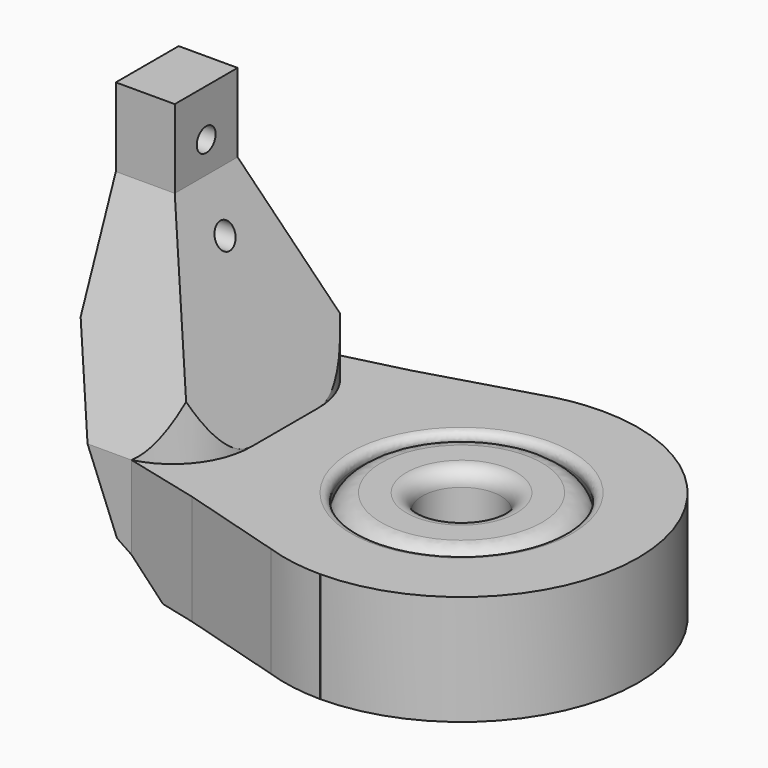
from build123d import *

# Parameters (mm, degrees)
F3_R         = 3
F4_R         = 1
F6_DEPTH     = 14
F7_T1_DEPTH  = 14
F8_DEPTH     = 10
F9_DEPTH     = 25
F10_W        = 50
F10_H        = 100
F11_DEPTH    = 50
F12_T1_DEPTH = 53.8936459138
F13_T1_DEPTH = 139.6556819565
F14_T4_DEPTH = 139.6556819565
F15_T1_DEPTH = 159.6556819565
F16_SIZE     = 5
F17_DEPTH    = 10
F18_R        = 1.5
F19_DEPTH    = 25
F20_R        = 2


# Not quite as in the source:
# - a fillet or chamfer that OpenCascade refuses, or shapes differently, is made with other operations: its cross-section is extruded or revolved along the edge and cut away or added


with BuildPart() as f2:
    # F0 (on Front) → F2 (revolve)
    with BuildSketch(Plane.XZ):
        with BuildLine():
            Line((5, 0), (12.124355653, 0))
            ThreePointArc((12.124355653, 0), (14, 7), (12.124355653, 14))
            Line((12.124355653, 14), (5, 14))
            Line((5, 14), (5, 0))
        make_face()
    revolve(axis=Axis((0, 0, 12.6064065844), (0, 0, 1)))

    # F3
    f3_edges = [f2.edges().sort_by_distance(p)[0] for p in [
        (-12.124356, 0, 14),
        (-12.124356, 0, 0),
    ]]
    fillet(f3_edges, radius=F3_R)

    # F20
    f20_edges = [f2.edges().sort_by_distance(p)[0] for p in [
        (-5, 0, 14),
    ]]
    fillet(f20_edges, radius=F20_R)


with BuildPart() as f2b:
    # F0 (on Front) → F2, piece 2 (revolve)
    with BuildSketch(Plane.XZ):
        with BuildLine():
            ThreePointArc((12.4695629434, 14), (14.3, 7), (12.4695629434, 0))
            Line((12.4695629434, 0), (22.4695629434, 0))
            Line((22.4695629434, 0), (22.4695629434, 14))
            Line((22.4695629434, 14), (12.4695629434, 14))
        make_face()
    revolve(axis=Axis((0, 0, 12.6064065844), (0, 0, 1)))

    # F4
    f4_edges = [f2b.edges().sort_by_distance(p)[0] for p in [
        (-12.469563, 0, 14),
        (-12.469563, 0, 0),
    ]]
    fillet(f4_edges, radius=F4_R)

    # F5 (on Top) → F6 (join)
    with BuildSketch(Plane.XY):
        Polygon((-15.7520063221, 9.0848943219), (0, 19.2215126008), (0, 22.5), (-30, 15), (-30, -15), (0, -22.5), (0, -18.8700128347), (-15.7520063221, -9.3158083037), align=None)
    extrude(amount=F6_DEPTH)

    # F7: chamfer of 20 on 2 edges, made by hand

    # F7_s2 → F7_t1 (join)
    with BuildSketch(Plane.XY):
        with BuildLine():
            Line((-6.4594864096, -21.5014925715), (-21.141510961, -17.1806268176))
            Line((-21.141510961, -17.1806268176), (-21.044496711, -16.7925698176))
            ThreePointArc((-21.044496711, -16.7925698176), (-15.7103098501, -18.1601119749), (-10.3681240616, -19.495658422))
            Line((-10.3681240616, -19.495658422), (-10.278839391, -19.5297483161))
            ThreePointArc((-10.278839391, -19.5297483161), (-8.3538564635, -20.4274004881), (-6.33083341, -21.1227467389))
            Line((-6.33083341, -21.1227467389), (-6.4594864096, -21.5014925715))
        make_face()
        with BuildLine():
            Line((-21.141510961, 17.1806268176), (-6.4594864096, 21.5014925715))
            Line((-6.4594864096, 21.5014925715), (-6.33083341, 21.1227467389))
            ThreePointArc((-6.33083341, 21.1227467389), (-8.3538564635, 20.4274004881), (-10.278839391, 19.5297483161))
            Line((-10.278839391, 19.5297483161), (-10.3681240616, 19.495658422))
            ThreePointArc((-10.3681240616, 19.495658422), (-15.7103098501, 18.1601119749), (-21.044496711, 16.7925698176))
            Line((-21.044496711, 16.7925698176), (-21.141510961, 17.1806268176))
        make_face()
    extrude(amount=F7_T1_DEPTH)

    # F8 (add): a face of the model
    f8_faces = [f2b.faces().sort_by_distance(p)[0] for p in [
        (-30, 0, 7),
    ]]
    extrude(f8_faces, amount=F8_DEPTH)

    # F9 (add): a face of the model
    f9_faces = [f2b.faces().sort_by_distance(p)[0] for p in [
        (21.6996638372, 0, 14),
    ]]
    extrude(f9_faces, amount=F9_DEPTH)

    # F10 (on Front) → F11 (cut, symmetric)
    with BuildSketch(Plane.XZ):
        with Locations((2.5, 64)):
            Rectangle(F10_W, F10_H)
    extrude(amount=F11_DEPTH, both=True, mode=Mode.SUBTRACT)

    # F12: fillet of radius 10 on 2 edges, made by hand

    # F12_s2 → F12_t1 (cut)
    with BuildSketch(Plane.XY.offset(14)):
        with BuildLine():
            ThreePointArc((-30, -15), (-24.5943058496, -11.4412659914), (-22.5, -5.3175416345))
            Line((-22.5, -5.3175416345), (-22.5, -16.875))
            Line((-22.5, -16.875), (-30, -15))
        make_face()
        with BuildLine():
            ThreePointArc((-22.5, 5.3175416345), (-24.5943058496, 11.4412659914), (-30, 15))
            Line((-30, 15), (-22.5, 16.875))
            Line((-22.5, 16.875), (-22.5, 5.3175416345))
        make_face()
    extrude(amount=F12_T1_DEPTH, mode=Mode.SUBTRACT)

    # F13: chamfer of 10 x 25 on 2 edges, made by hand

    # F13_s2 → F13_t1 (cut)
    with BuildSketch(Plane.YZ.offset(-104.8278409783)):
        Polygon((-15, 14), (-5, 39), (-15, 39), align=None)
        Polygon((15, 14), (5, 39), (15, 39), align=None)
    extrude(amount=F13_T1_DEPTH, mode=Mode.SUBTRACT)

    # F14: chamfer of 25 x 10 on 1 edges, made by hand


with BuildPart() as f14_tool2:
    # F14_s3 → F14_t4 (new body)
    with BuildSketch(Plane.XZ.offset(-69.8278409783)):
        Polygon((-22.5, 14), (-32.5, 39), (-22.5, 39), align=None)
    extrude(amount=F14_T4_DEPTH)

    split(bisect_by=Plane.XY.offset(14), keep=Keep.TOP)


with BuildPart() as f2b_1:
    add(f2b.part)

    # F14_t1: cut F14_tool2
    add(f14_tool2.part, mode=Mode.SUBTRACT)

    # F15: chamfer of 10 x 25 on 1 edges, made by hand

    # F15_s2 → F15_t1 (cut)
    with BuildSketch(Plane.XZ.offset(-79.8278409783)):
        Polygon((-40, 25), (-30, 0), (-40, 0), align=None)
    extrude(amount=F15_T1_DEPTH, mode=Mode.SUBTRACT)

    # F16
    f16_edges = [f2b_1.edges().sort_by_distance(p)[0] for p in [
        (-30, 0, 0),
    ]]
    chamfer(f16_edges, length=F16_SIZE)

    # F17 (add): a face of the model
    f17_faces = [f2b_1.faces().sort_by_distance(p)[0] for p in [
        (-36.25, 0, 39),
    ]]
    extrude(f17_faces, amount=F17_DEPTH)

    # F18 (on face) → F19 (cut)
    with BuildSketch(Plane(origin=(-40, 0, 0), x_dir=(0, -1, 0), z_dir=(-1, 0, 0))):
        with Locations((0, 33)):
            Circle(F18_R)
        with Locations((0, 43)):
            Circle(F18_R)
    extrude(amount=-F19_DEPTH, mode=Mode.SUBTRACT)


solid = Compound([f2.part, f2b_1.part])
